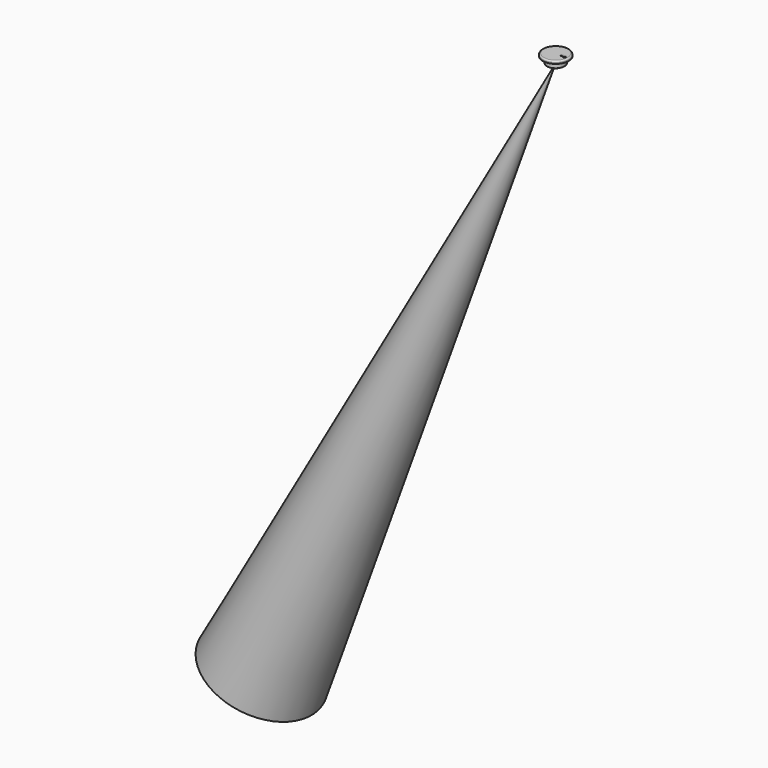
from build123d import *

# Parameters (mm, degrees)
F2_W     = 100
F2_H     = 70
F4_R     = 15
F7_DEPTH = 2


# Not quite as in the source:
# - a feature names something its author has since deleted; it is built from what else it names


with BuildPart() as f1:
    # F0 (on Front) → F1 (revolve)
    with BuildSketch(Plane.XZ):
        with BuildLine():
            Line((-3380.9460939256, -7250.4622962932), (0, 0))
            Line((0, 0), (-24.6211780052, -43.517784797))
            Line((-24.6211780052, -43.517784797), (-1969.6942404139, -3481.4227837596))
            Line((-1969.6942404139, -3481.4227837596), (-2462.1178005173, -4351.7784796995))
            Line((-2462.1178005173, -4351.7784796995), (-3446.9649207243, -6092.4898715793))
            Line((-3446.9649207243, -6092.4898715793), (-3939.3884808277, -6962.8455675192))
            ThreePointArc((-3939.3884808277, -6962.8455675192), (-3662.9913209357, -7112.1371318859), (-3380.9460939256, -7250.4622962932))
        make_face()
        with BuildLine():
            Line((-24.6211780052, -43.517784797), (0, 0))
            Line((0, 0), (21.130913087, 45.3153893518))
            ThreePointArc((21.130913087, 45.3153893518), (-44.4508570743, 22.8936957558), (-24.6211780052, -43.517784797))
        make_face()
    revolve(axis=Axis((-1690.4730469628, 0, -3625.2311481466), (-0.4226182617, 0, -0.906307787)))


with BuildPart() as f3:
    # F2 (on Right) → F3 (revolve)
    with BuildSketch(Plane.YZ):
        with Locations((-50, 35)):
            Rectangle(F2_W, F2_H)
        Polygon((-100, 70), (0, 70), (0, 100), (-150, 100), (-150, 70), align=None)
    revolve(axis=Axis((0, 0, 35), (0, 0, 1)))

    # F4
    f4_edges = [f3.edges().sort_by_distance(p)[0] for p in [
        (0, 150, 100),
    ]]
    fillet(f4_edges, radius=F4_R)

    # F6 (on offset) → F7 (join)
    with BuildSketch(Plane.XY.offset(100)):
        Polygon((102.5, -20), (132.5, 0), (102.5, 20), (102.5, 10), (62.5, 10), (62.5, 0), (62.5, -10), (102.5, -10), align=None)
    extrude(amount=F7_DEPTH)


solid = Compound([f1.part, f3.part])
